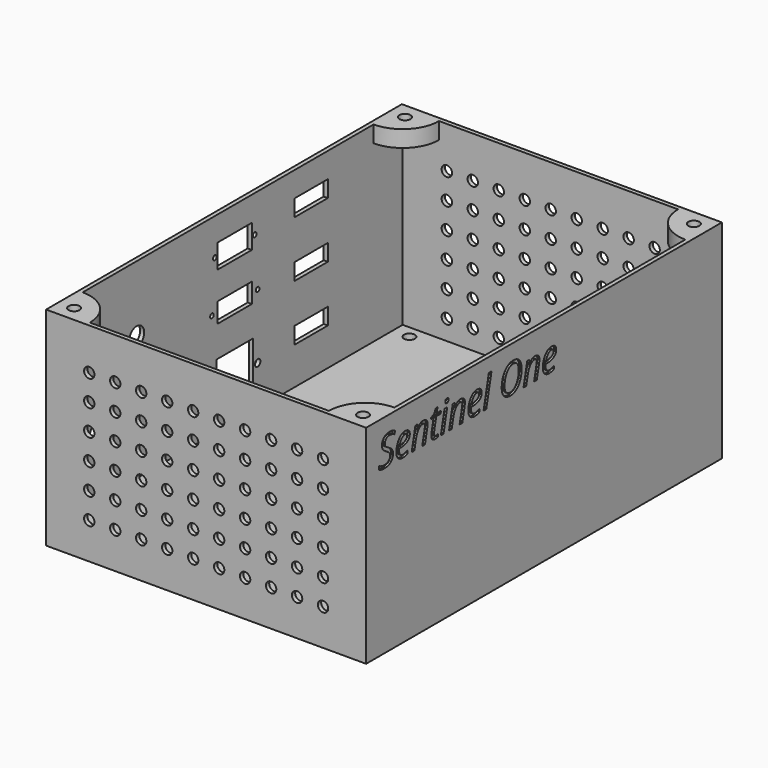
from build123d import *

# Parameters (mm, degrees)
F0_W           = 150
F0_H           = 210
F1_DEPTH       = 8
F0_W_2         = 154
F0_H_2         = 214
F2_DEPTH       = 100
F3_W           = 20.5
F3_H           = 11.5
F3_W_2         = 22
F3_H_2         = 23
F3_W_3         = 20
F3_H_3         = 8
F3_H_4         = 9.5
F3_R           = 4.5
F4_DEPTH       = 2
F6_D           = 2.2
F6_DEPTH       = 5
F6_TIP         = 0.6609466809
F7_D           = 3.3
F7_DEPTH       = 5
F7_TIP         = 0.9914200214
F8_TEXT_SIZE   = 1.8718102452
F8_TEXT_SIZE_2 = 2.0222766411
F8_TEXT_SIZE_3 = 3.0363412088
F8_TEXT_SIZE_4 = 2.4859058019
F8_TEXT_SIZE_5 = 2.7080613182
F8_TEXT_SIZE_6 = 2.8339901696
F8_TEXT_SIZE_7 = 2.0882276168
F8_TEXT_SIZE_8 = 2.6374350944
F9_DEPTH       = 1
F10_R          = 2.65
F11_DEPTH      = 6.2
F12_TEXT_SIZE  = 19.4444444444
F13_DEPTH      = 1
F3_R_2         = 3.5
F14_DEPTH      = 2
F16_DEPTH      = 8
F17_R          = 2.5
F18_DEPTH      = 2
F19_R          = 2.5
F20_DEPTH      = 2
F21_R          = 2.65
F22_DEPTH      = 6.2


# Not quite as in the source:
# - a feature names something its author has since deleted; it is built from what else it names
# - Text() gives the source's letters only with a copy of the font that has no kerning and outlines rounded to 1/6400 em; it was checked with that copy


with BuildPart() as f1:
    # F0 (on Top) → F1 (new body)
    with BuildSketch(Plane.XY):
        Rectangle(F0_W, F0_H)
    extrude(amount=F1_DEPTH)

    # F0 (on Top) → F2 (join)
    with BuildSketch(Plane.XY):
        Rectangle(F0_W_2, F0_H_2)
        Rectangle(F0_W, F0_H, mode=Mode.SUBTRACT)
    extrude(amount=F2_DEPTH)

    # F3 (on face) → F4 (cut, through all)
    with BuildSketch(Plane.YZ.offset(-75)):
        with Locations((4, 82.3520267606)):
            Rectangle(F3_W, F3_H)
        with Locations((4, 27.32265459)):
            Rectangle(F3_W_2, F3_H_2)
        with Locations((49.95, 30)):
            Rectangle(F3_W_3, F3_H_3)
        with Locations((49.95, 57)):
            Rectangle(F3_W_3, F3_H_3)
        with Locations((49.95, 84)):
            Rectangle(F3_W_3, F3_H_3)
        with Locations((4, 58.4434465468)):
            Rectangle(F3_W, F3_H_4)
        with Locations((-55, 68)):
            Circle(F3_R)
    extrude(amount=-F4_DEPTH, mode=Mode.SUBTRACT)

    # F6
    with Locations(Plane(origin=(-77, 0, 0), x_dir=(0, -1, 0), z_dir=(-1, 0, 0))):
        with Locations((-16, 82.3520267606), (8, 82.3520267606), (-17.75, 58.4434465468), (9.75, 58.4434465468)):
            Hole(F6_D / 2, depth=F6_DEPTH)
            with Locations((0, 0, -(F6_DEPTH + F6_TIP / 2))):  # 118° drill point
                Cone(0, F6_D / 2, F6_TIP, mode=Mode.SUBTRACT)

    # F7
    with Locations(Plane(origin=(-77, 0, 0), x_dir=(0, -1, 0), z_dir=(-1, 0, 0))):
        with Locations((9.75, 27.32265459), (-17.75, 27.32265459)):
            Hole(F7_D / 2, depth=F7_DEPTH)
            with Locations((0, 0, -(F7_DEPTH + F7_TIP / 2))):  # 118° drill point
                Cone(0, F7_D / 2, F7_TIP, mode=Mode.SUBTRACT)

    # F8 (on face) → F9 (cut)
    with BuildSketch(Plane(origin=(-77, 0, 0), x_dir=(0, -1, 0), z_dir=(-1, 0, 0))):
        with Locations((-59.95, 76.6522966234)):
            Text('FRONT CAMERA INPUT', F8_TEXT_SIZE, font='Open Sans', text_align=(TextAlign.LEFT, TextAlign.BOTTOM))
        with Locations((-59.95, 22.5439608184)):
            Text('REAR CAMERA INPUT', F8_TEXT_SIZE_2, font='Open Sans', text_align=(TextAlign.LEFT, TextAlign.BOTTOM))
        with Locations((-11.5, 11.6364889196)):
            Text('ETHERNET', F8_TEXT_SIZE_3, font='Open Sans', text_align=(TextAlign.LEFT, TextAlign.BOTTOM))
        with Locations((-12.75, 49.9035943694)):
            Text('MONITOR OUT', F8_TEXT_SIZE_4, font='Open Sans', text_align=(TextAlign.LEFT, TextAlign.BOTTOM))
        with Locations((-12.75, 72.6522226114)):
            Text('RADAR INPUT', F8_TEXT_SIZE_5, font='Open Sans', text_align=(TextAlign.LEFT, TextAlign.BOTTOM))
        with Locations((50, 59.4595270779)):
            Text('POWER', F8_TEXT_SIZE_6, font='Open Sans', text_align=(TextAlign.LEFT, TextAlign.BOTTOM))
        with Locations((-59.95, 49.4964761159)):
            Text('SIDE CAMERA INPUT', F8_TEXT_SIZE_7, font='Open Sans', text_align=(TextAlign.LEFT, TextAlign.BOTTOM))
        with Locations((77, 30.6010467321)):
            Text('GPS', F8_TEXT_SIZE_8, font='Open Sans', text_align=(TextAlign.LEFT, TextAlign.BOTTOM))
    extrude(amount=-F9_DEPTH, mode=Mode.SUBTRACT)

    # F10 (on face) → F11 (cut)
    with BuildSketch(Plane.XY.offset(8)):
        with Locations((-66.95, 99)):
            Circle(F10_R)
        with Locations((-66.95, 30)):
            Circle(F10_R)
        with Locations((13.95, 30)):
            Circle(F10_R)
        with Locations((13.95, 99)):
            Circle(F10_R)
        with Locations((-67.5, -30.5)):
            Circle(F10_R)
        with Locations((66.5, -30.5)):
            Circle(F10_R)
        with Locations((65.5, -96.5)):
            Circle(F10_R)
        with Locations((-66.5, -96.5)):
            Circle(F10_R)
    extrude(amount=-F11_DEPTH, mode=Mode.SUBTRACT)

    # F12 (on face) → F13 (cut)
    with BuildSketch(Plane.YZ.offset(77)):
        with Locations((-99.5, 78.5)):
            Text('Sentinel One', F12_TEXT_SIZE, font='Open Sans', font_style=FontStyle.ITALIC, text_align=(TextAlign.LEFT, TextAlign.BOTTOM))
    extrude(amount=-F13_DEPTH, mode=Mode.SUBTRACT)

    # F3 (on face) → F14 (cut, through all)
    with BuildSketch(Plane.YZ.offset(-75)):
        with Locations((-79.5, 38)):
            Circle(F3_R_2)
    extrude(amount=-F14_DEPTH, mode=Mode.SUBTRACT)

    # F15 (on face) → F16 (join)
    with BuildSketch(Plane.XY.offset(100)):
        with BuildLine():
            ThreePointArc((-75, 87.5), (-62.6256313292, 92.6256313292), (-57.5, 105))
            Line((-57.5, 105), (-75, 105))
            Line((-75, 105), (-75, 87.5))
        make_face()
        with BuildLine():
            Line((75, 105), (57.5, 105))
            ThreePointArc((57.5, 105), (62.6256313292, 92.6256313292), (75, 87.5))
            Line((75, 87.5), (75, 105))
        make_face()
        with BuildLine():
            Line((75, -105), (75, -87.5))
            ThreePointArc((75, -87.5), (62.6256313292, -92.6256313292), (57.5, -105))
            Line((57.5, -105), (75, -105))
        make_face()
        with BuildLine():
            ThreePointArc((-57.5, -105), (-62.6256313292, -92.6256313292), (-75, -87.5))
            Line((-75, -87.5), (-75, -105))
            Line((-75, -105), (-57.5, -105))
        make_face()
    extrude(amount=-F16_DEPTH)

    # F17 (on face) → F18 (cut, through all)
    with BuildSketch(Plane.XZ.offset(107)):
        with Locations((-6.225, 42.5)):
            Circle(F17_R)
        with Locations((-43.725, 17.5)):
            Circle(F17_R)
        with Locations((6.275, 17.5)):
            Circle(F17_R)
        with Locations((18.775, 80)):
            Circle(F17_R)
        with Locations((18.775, 30)):
            Circle(F17_R)
        with Locations((-56.225, 17.5)):
            Circle(F17_R)
        with Locations((31.275, 55)):
            Circle(F17_R)
        with Locations((31.275, 17.5)):
            Circle(F17_R)
        with Locations((18.775, 17.5)):
            Circle(F17_R)
        with Locations((18.775, 67.5)):
            Circle(F17_R)
        with Locations((-31.225, 42.5)):
            Circle(F17_R)
        with Locations((-56.225, 30)):
            Circle(F17_R)
        with Locations((43.775, 42.5)):
            Circle(F17_R)
        with Locations((-6.225, 30)):
            Circle(F17_R)
        with Locations((18.775, 42.5)):
            Circle(F17_R)
        with Locations((6.275, 67.5)):
            Circle(F17_R)
        with Locations((31.275, 67.5)):
            Circle(F17_R)
        with Locations((6.275, 80)):
            Circle(F17_R)
        with Locations((-31.225, 30)):
            Circle(F17_R)
        with Locations((-31.225, 17.5)):
            Circle(F17_R)
        with Locations((-18.725, 42.5)):
            Circle(F17_R)
        with Locations((-18.725, 30)):
            Circle(F17_R)
        with Locations((56.275, 30)):
            Circle(F17_R)
        with Locations((31.275, 80)):
            Circle(F17_R)
        with Locations((6.275, 55)):
            Circle(F17_R)
        with Locations((-43.725, 42.5)):
            Circle(F17_R)
        with Locations((-6.225, 55)):
            Circle(F17_R)
        with Locations((18.775, 55)):
            Circle(F17_R)
        with Locations((56.275, 17.5)):
            Circle(F17_R)
        with Locations((-56.225, 42.5)):
            Circle(F17_R)
        with Locations((43.775, 55)):
            Circle(F17_R)
        with Locations((-6.225, 17.5)):
            Circle(F17_R)
        with Locations((43.775, 17.5)):
            Circle(F17_R)
        with Locations((31.275, 30)):
            Circle(F17_R)
        with Locations((31.275, 42.5)):
            Circle(F17_R)
        with Locations((56.275, 42.5)):
            Circle(F17_R)
        with Locations((-18.725, 17.5)):
            Circle(F17_R)
        with Locations((6.275, 42.5)):
            Circle(F17_R)
        with Locations((-43.725, 30)):
            Circle(F17_R)
        with Locations((43.775, 30)):
            Circle(F17_R)
        with Locations((6.275, 30)):
            Circle(F17_R)
        with Locations((-31.225, 67.5)):
            Circle(F17_R)
        with Locations((56.275, 67.5)):
            Circle(F17_R)
        with Locations((-31.225, 55)):
            Circle(F17_R)
        with Locations((-43.725, 55)):
            Circle(F17_R)
        with Locations((56.275, 55)):
            Circle(F17_R)
        with Locations((-43.725, 67.5)):
            Circle(F17_R)
        with Locations((-6.225, 67.5)):
            Circle(F17_R)
        with Locations((56.275, 80)):
            Circle(F17_R)
        with Locations((-18.725, 80)):
            Circle(F17_R)
        with Locations((-18.725, 55)):
            Circle(F17_R)
        with Locations((-18.725, 67.5)):
            Circle(F17_R)
        with Locations((43.775, 67.5)):
            Circle(F17_R)
        with Locations((-56.225, 80)):
            Circle(F17_R)
        with Locations((-6.225, 80)):
            Circle(F17_R)
        with Locations((-31.225, 80)):
            Circle(F17_R)
        with Locations((-56.225, 55)):
            Circle(F17_R)
        with Locations((-56.225, 67.5)):
            Circle(F17_R)
        with Locations((43.775, 80)):
            Circle(F17_R)
        with Locations((-43.725, 80)):
            Circle(F17_R)
    extrude(amount=-F18_DEPTH, mode=Mode.SUBTRACT)

    # F19 (on face) → F20 (cut, through all)
    with BuildSketch(Plane(origin=(0, 107, 0), x_dir=(-1, 0, 0), z_dir=(0, 1, 0))):
        with Locations((28.775, 55)):
            Circle(F19_R)
        with Locations((28.775, 80)):
            Circle(F19_R)
        with Locations((-58.725, 30)):
            Circle(F19_R)
        with Locations((3.775, 55)):
            Circle(F19_R)
        with Locations((3.775, 67.5)):
            Circle(F19_R)
        with Locations((-58.725, 17.5)):
            Circle(F19_R)
        with Locations((53.775, 80)):
            Circle(F19_R)
        with Locations((-21.225, 67.5)):
            Circle(F19_R)
        with Locations((-46.225, 42.5)):
            Circle(F19_R)
        with Locations((53.775, 17.5)):
            Circle(F19_R)
        with Locations((-8.725, 67.5)):
            Circle(F19_R)
        with Locations((-33.725, 42.5)):
            Circle(F19_R)
        with Locations((-8.725, 17.5)):
            Circle(F19_R)
        with Locations((3.775, 80)):
            Circle(F19_R)
        with Locations((-33.725, 30)):
            Circle(F19_R)
        with Locations((-58.725, 55)):
            Circle(F19_R)
        with Locations((53.775, 30)):
            Circle(F19_R)
        with Locations((41.275, 30)):
            Circle(F19_R)
        with Locations((28.775, 30)):
            Circle(F19_R)
        with Locations((-46.225, 80)):
            Circle(F19_R)
        with Locations((41.275, 42.5)):
            Circle(F19_R)
        with Locations((16.275, 67.5)):
            Circle(F19_R)
        with Locations((16.275, 55)):
            Circle(F19_R)
        with Locations((-8.725, 80)):
            Circle(F19_R)
        with Locations((41.275, 17.5)):
            Circle(F19_R)
        with Locations((28.775, 42.5)):
            Circle(F19_R)
        with Locations((-21.225, 80)):
            Circle(F19_R)
        with Locations((-46.225, 55)):
            Circle(F19_R)
        with Locations((41.275, 80)):
            Circle(F19_R)
        with Locations((53.775, 67.5)):
            Circle(F19_R)
        with Locations((-46.225, 67.5)):
            Circle(F19_R)
        with Locations((-8.725, 30)):
            Circle(F19_R)
        with Locations((3.775, 30)):
            Circle(F19_R)
        with Locations((-8.725, 42.5)):
            Circle(F19_R)
        with Locations((16.275, 30)):
            Circle(F19_R)
        with Locations((16.275, 42.5)):
            Circle(F19_R)
        with Locations((-33.725, 67.5)):
            Circle(F19_R)
        with Locations((16.275, 17.5)):
            Circle(F19_R)
        with Locations((41.275, 55)):
            Circle(F19_R)
        with Locations((53.775, 42.5)):
            Circle(F19_R)
        with Locations((3.775, 17.5)):
            Circle(F19_R)
        with Locations((-58.725, 67.5)):
            Circle(F19_R)
        with Locations((28.775, 67.5)):
            Circle(F19_R)
        with Locations((28.775, 17.5)):
            Circle(F19_R)
        with Locations((-58.725, 42.5)):
            Circle(F19_R)
        with Locations((-58.725, 80)):
            Circle(F19_R)
        with Locations((16.275, 80)):
            Circle(F19_R)
        with Locations((3.775, 42.5)):
            Circle(F19_R)
        with Locations((-21.225, 55)):
            Circle(F19_R)
        with Locations((41.275, 67.5)):
            Circle(F19_R)
        with Locations((-21.225, 17.5)):
            Circle(F19_R)
        with Locations((53.775, 55)):
            Circle(F19_R)
        with Locations((-33.725, 17.5)):
            Circle(F19_R)
        with Locations((-21.225, 30)):
            Circle(F19_R)
        with Locations((-46.225, 17.5)):
            Circle(F19_R)
        with Locations((-33.725, 55)):
            Circle(F19_R)
        with Locations((-21.225, 42.5)):
            Circle(F19_R)
        with Locations((-46.225, 30)):
            Circle(F19_R)
        with Locations((-33.725, 80)):
            Circle(F19_R)
        with Locations((-8.725, 55)):
            Circle(F19_R)
    extrude(amount=-F20_DEPTH, mode=Mode.SUBTRACT)

    # F21 (on face) → F22 (cut)
    with BuildSketch(Plane.XY.offset(100)):
        with Locations((69.5, -99.5)):
            Circle(F21_R)
        with Locations((-69.5, -99.5)):
            Circle(F21_R)
        with Locations((-69.5, 99.5)):
            Circle(F21_R)
        with Locations((69.5, 99.5)):
            Circle(F21_R)
    extrude(amount=-F22_DEPTH, mode=Mode.SUBTRACT)


solid = f1.part
